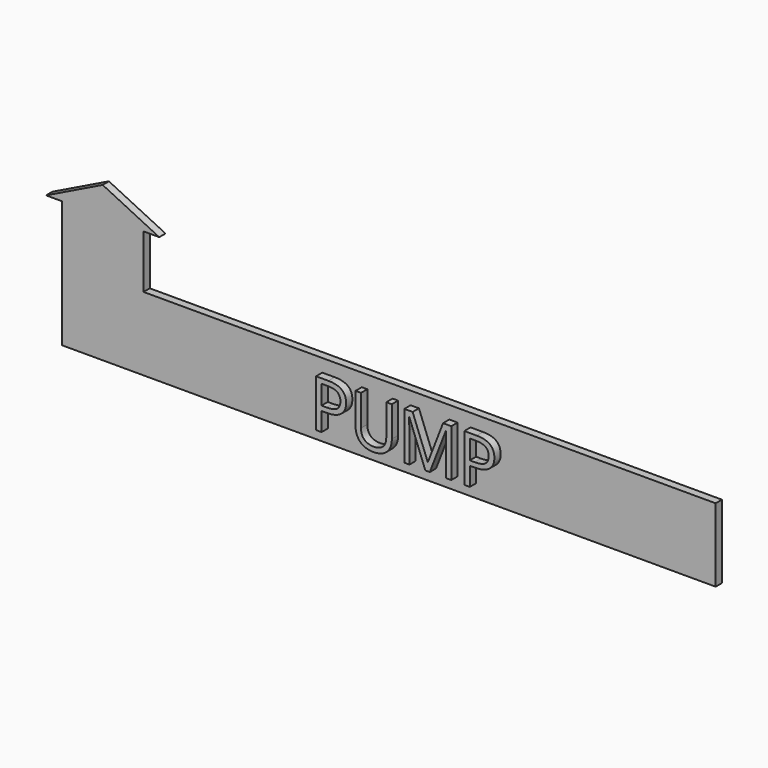
from build123d import *

# Parameters (mm, degrees)
F1_DEPTH     = 25
F2_TEXT_SIZE = 210.9920088616
F3_DEPTH     = 25


# Not quite as in the source:
# - Text() gives the source's letters only with a copy of the font that has no kerning and outlines rounded to 1/6400 em; it was checked with that copy


with BuildPart() as f1:
    # F0 (on Front) → F1 (new body)
    with BuildSketch(Plane.XZ):
        Polygon((-2046.8193110937, 286.6455302747), (-2046.8193110937, 45.6370309986), (30.593802718, 45.6370309986), (30.593802718, 279.0184617043), (-1787.301692574, 279.0184617043), (-1787.301692574, 448.4629034996), (-1737.301692574, 448.4629034996), (-1917.0605018339, 536.1371328574), (-2096.8193110937, 448.4629034996), (-2046.8193110937, 448.4629034996), align=None)
    extrude(amount=-F1_DEPTH)


with BuildPart() as f3:
    # F2 (on Front) → F3 (new body)
    with BuildSketch(Plane.XZ):
        with Locations((-1239.8025095463, 87.4781385064)):
            Text('PUMP', F2_TEXT_SIZE, font='Open Sans', text_align=(TextAlign.LEFT, TextAlign.BOTTOM))
    extrude(amount=F3_DEPTH)


solid = Compound([f1.part, f3.part])
